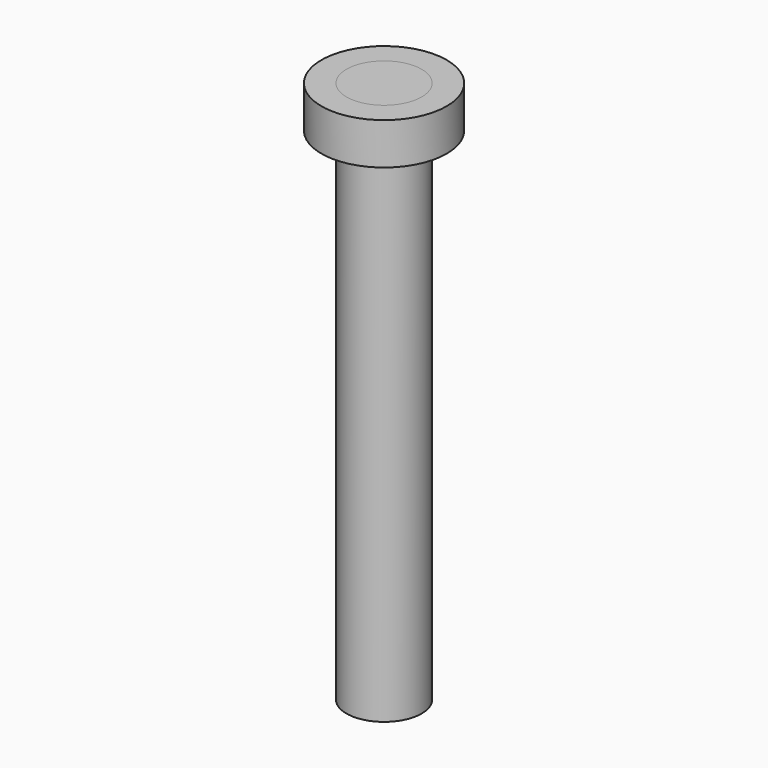
from build123d import *

# Parameters (mm, degrees)
F0_R     = 0.9
F1_DEPTH = 12
F0_R_2   = 1.5
F2_DEPTH = 1
F3_DEPTH = 1


with BuildPart() as f1:
    # F0 (on Top) → F1 (new body)
    with BuildSketch(Plane.XY):
        Circle(F0_R)
    extrude(amount=-F1_DEPTH)

    # F3 (add, through all): a face of the model
    f3_faces = [f1.faces().sort_by_distance(p)[0] for p in [
        (0, 0, 0),
    ]]
    extrude(f3_faces, amount=F3_DEPTH)


with BuildPart() as f2:
    # F0 (on Top) → F2 (new body)
    with BuildSketch(Plane.XY):
        Circle(F0_R_2)
        Circle(F0_R, mode=Mode.SUBTRACT)
    extrude(amount=F2_DEPTH)


solid = Compound([f1.part, f2.part])
